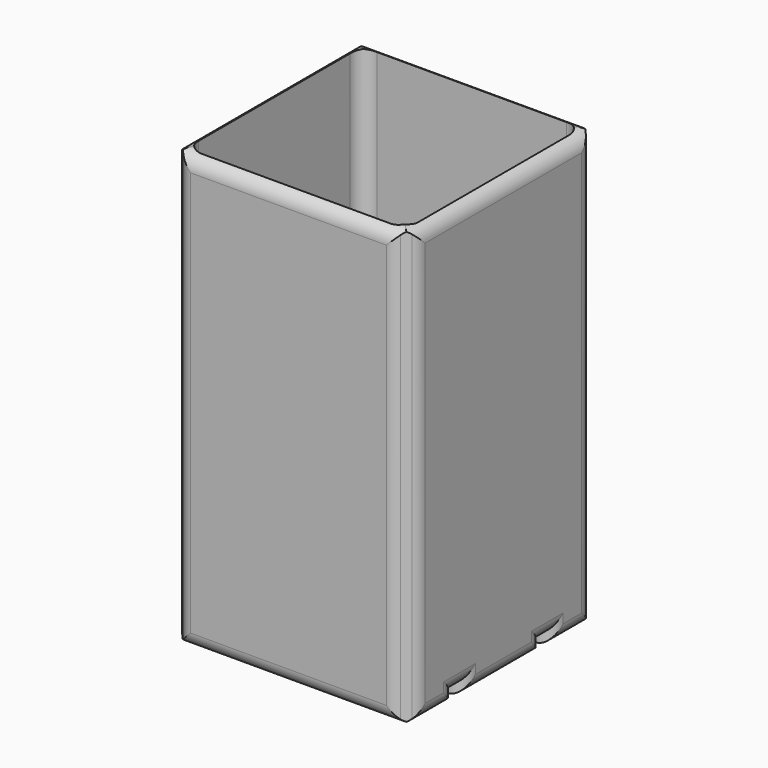
from build123d import *

# Parameters (mm, degrees)
F0_W         = 80.0557104707
F0_H         = 80.0557104707
F0_W_2       = 73.7057104707
F0_H_2       = 73.7057104707
F0_W_3       = 39.99992
F0_H_3       = 39.99992
F1_DEPTH     = 6.35
F2_DEPTH     = 9.144
F3_DEPTH     = 139.7
F4_W         = 20.0278952353
F4_H         = 3.175
F5_DEPTH     = 3.175
F6_SIZE      = 5.08
F7_T1_DEPTH  = 95.2957104707
F7_T3_DEPTH  = 156.5710244843
F7_T5_DEPTH  = 95.2957104707
F7_T7_DEPTH  = 40.3478952353
F7_T9_DEPTH  = 40.3478952353
F7_T11_DEPTH = 15.875
F7_T13_DEPTH = 3.175
F7_T15_DEPTH = 3.175
F7_T17_DEPTH = 59.04992
F7_T23_DEPTH = 28.575
F7_T27_DEPTH = 15.875
F7_T34_DEPTH = 28.575
F7_T38_DEPTH = 15.875
F7_T45_DEPTH = 15.875
F7_T49_DEPTH = 28.575
F7_T56_DEPTH = 15.875
F7_T60_DEPTH = 28.575
F8_R         = 5.08


# Not quite as in the source:
# - a fillet or chamfer that OpenCascade refuses, or shapes differently, is made with other operations: its cross-section is extruded or revolved along the edge and cut away or added


with BuildPart() as f1:
    # F0 (on Top) → F1 (new body)
    with BuildSketch(Plane.XY):
        Rectangle(F0_W, F0_H)
        Rectangle(F0_W_2, F0_H_2, mode=Mode.SUBTRACT)
        Rectangle(F0_W_2, F0_H_2)
        Rectangle(F0_W_3, F0_H_3, mode=Mode.SUBTRACT)
        Rectangle(F0_W_3, F0_H_3)
    extrude(amount=-F1_DEPTH)

    # F0 (on Top) → F2 (cut)
    with BuildSketch(Plane.XY):
        Rectangle(F0_W_3, F0_H_3)
    extrude(amount=-F2_DEPTH, mode=Mode.SUBTRACT)

    # F0 (on Top) → F3 (join)
    with BuildSketch(Plane.XY):
        Rectangle(F0_W, F0_H)
        Rectangle(F0_W_2, F0_H_2, mode=Mode.SUBTRACT)
    extrude(amount=F3_DEPTH)

    # F4 (on face) → F5 (cut)
    with BuildSketch(Plane(origin=(0, 0, -6.35), x_dir=(1, 0, 0), z_dir=(0, 0, -1))):
        with Locations((30.0139076177, 18.41246)):
            Rectangle(F4_W, F4_H)
        with Locations((30.0139076177, -18.41246)):
            Rectangle(F4_W, F4_H)
    extrude(amount=-F5_DEPTH, mode=Mode.SUBTRACT)

    # F6
    f6_edges = [f1.edges().sort_by_distance(p)[0] for p in [
        (40.027855, -40.027855, 66.675),
        (-40.027855, -40.027855, 66.675),
        (-40.027855, 40.027855, 66.675),
        (40.027855, 40.027855, 66.675),
    ]]
    chamfer(f6_edges, length=F6_SIZE)

    # F7: fillet of radius 5.08 on 24 edges, made by hand

    # F7_s2 → F7_t1 (cut)
    with BuildSketch(Plane.XZ.offset(-47.6478552353)):
        with BuildLine():
            ThreePointArc((-34.9478552353, -6.35), (-38.5399576838, -4.8621024484), (-40.0278552353, -1.27))
            Line((-40.0278552353, -1.27), (-40.0278552353, -6.35))
            Line((-40.0278552353, -6.35), (-34.9478552353, -6.35))
        make_face()
        with BuildLine():
            ThreePointArc((-34.9478552353, 139.7), (-38.5399576838, 138.2121024484), (-40.0278552353, 134.62))
            Line((-40.0278552353, 134.62), (-40.0278552353, 139.7))
            Line((-40.0278552353, 139.7), (-34.9478552353, 139.7))
        make_face()
        with BuildLine():
            ThreePointArc((40.0278552353, 134.62), (38.5399576838, 138.2121024484), (34.9478552353, 139.7))
            Line((34.9478552353, 139.7), (40.0278552353, 139.7))
            Line((40.0278552353, 139.7), (40.0278552353, 134.62))
        make_face()
    extrude(amount=F7_T1_DEPTH, mode=Mode.SUBTRACT)

    # F7_s4 → F7_t3 (cut)
    with BuildSketch(Plane.XY.offset(-11.6105122421)):
        with BuildLine():
            ThreePointArc((-38.5399576838, 36.4357527869), (-39.6411632605, 34.7876821749), (-40.0278552353, 32.8436503385))
            Line((-40.0278552353, 32.8436503385), (-40.0278552353, 34.9478552353))
            Line((-40.0278552353, 34.9478552353), (-38.5399576838, 36.4357527869))
        make_face()
        with BuildLine():
            ThreePointArc((-38.5399576838, -36.4357527869), (-39.6411632605, -34.7876821749), (-40.0278552353, -32.8436503385))
            Line((-40.0278552353, -32.8436503385), (-40.0278552353, -34.9478552353))
            Line((-40.0278552353, -34.9478552353), (-38.5399576838, -36.4357527869))
        make_face()
        with BuildLine():
            ThreePointArc((36.4357527869, 38.5399576838), (34.7876821749, 39.6411632605), (32.8436503385, 40.0278552353))
            Line((32.8436503385, 40.0278552353), (34.9478552353, 40.0278552353))
            Line((34.9478552353, 40.0278552353), (36.4357527869, 38.5399576838))
        make_face()
        with BuildLine():
            ThreePointArc((-32.8436503385, 40.0278552353), (-34.7876821749, 39.6411632605), (-36.4357527869, 38.5399576838))
            Line((-36.4357527869, 38.5399576838), (-34.9478552353, 40.0278552353))
            Line((-34.9478552353, 40.0278552353), (-32.8436503385, 40.0278552353))
        make_face()
        with BuildLine():
            ThreePointArc((40.0278552353, -32.8436503385), (39.6411632605, -34.7876821749), (38.5399576838, -36.4357527869))
            Line((38.5399576838, -36.4357527869), (40.0278552353, -34.9478552353))
            Line((40.0278552353, -34.9478552353), (40.0278552353, -32.8436503385))
        make_face()
        with BuildLine():
            ThreePointArc((40.0278552353, 32.8436503385), (39.6411632605, 34.7876821749), (38.5399576838, 36.4357527869))
            Line((38.5399576838, 36.4357527869), (40.0278552353, 34.9478552353))
            Line((40.0278552353, 34.9478552353), (40.0278552353, 32.8436503385))
        make_face()
        with BuildLine():
            ThreePointArc((-32.8436503385, -40.0278552353), (-34.7876821749, -39.6411632605), (-36.4357527869, -38.5399576838))
            Line((-36.4357527869, -38.5399576838), (-34.9478552353, -40.0278552353))
            Line((-34.9478552353, -40.0278552353), (-32.8436503385, -40.0278552353))
        make_face()
        with BuildLine():
            ThreePointArc((36.4357527869, -38.5399576838), (34.7876821749, -39.6411632605), (32.8436503385, -40.0278552353))
            Line((32.8436503385, -40.0278552353), (34.9478552353, -40.0278552353))
            Line((34.9478552353, -40.0278552353), (36.4357527869, -38.5399576838))
        make_face()
    extrude(amount=F7_T3_DEPTH, mode=Mode.SUBTRACT)

    # F7_s6 → F7_t5 (cut)
    with BuildSketch(Plane.YZ.offset(-47.6478552353)):
        with BuildLine():
            ThreePointArc((34.9478552353, -6.35), (38.5399576838, -4.8621024484), (40.0278552353, -1.27))
            Line((40.0278552353, -1.27), (40.0278552353, -6.35))
            Line((40.0278552353, -6.35), (34.9478552353, -6.35))
        make_face()
        with BuildLine():
            ThreePointArc((34.9478552353, 139.7), (38.5399576838, 138.2121024484), (40.0278552353, 134.62))
            Line((40.0278552353, 134.62), (40.0278552353, 139.7))
            Line((40.0278552353, 139.7), (34.9478552353, 139.7))
        make_face()
        with BuildLine():
            ThreePointArc((-34.9478552353, -6.35), (-38.5399576838, -4.8621024484), (-40.0278552353, -1.27))
            Line((-40.0278552353, -1.27), (-40.0278552353, -6.35))
            Line((-40.0278552353, -6.35), (-34.9478552353, -6.35))
        make_face()
        with BuildLine():
            ThreePointArc((-34.9478552353, 139.7), (-38.5399576838, 138.2121024484), (-40.0278552353, 134.62))
            Line((-40.0278552353, 134.62), (-40.0278552353, 139.7))
            Line((-40.0278552353, 139.7), (-34.9478552353, 139.7))
        make_face()
    extrude(amount=F7_T5_DEPTH, mode=Mode.SUBTRACT)

    # F7_s8 → F7_t7 (cut)
    with BuildSketch(Plane.XZ.offset(7.29996)):
        with BuildLine():
            ThreePointArc((40.0278552353, -1.27), (38.5399576838, -4.8621024484), (34.9478552353, -6.35))
            Line((34.9478552353, -6.35), (40.0278552353, -6.35))
            Line((40.0278552353, -6.35), (40.0278552353, -1.27))
        make_face()
    extrude(amount=F7_T7_DEPTH, mode=Mode.SUBTRACT)

    # F7_s10 → F7_t9 (cut)
    with BuildSketch(Plane.XZ.offset(-47.6478552353)):
        with BuildLine():
            ThreePointArc((40.0278552353, -1.27), (38.5399576838, -4.8621024484), (34.9478552353, -6.35))
            Line((34.9478552353, -6.35), (40.0278552353, -6.35))
            Line((40.0278552353, -6.35), (40.0278552353, -1.27))
        make_face()
    extrude(amount=F7_T9_DEPTH, mode=Mode.SUBTRACT)

    # F7_s12 → F7_t11 (cut)
    with BuildSketch(Plane.XY.offset(-19.05)):
        with BuildLine():
            ThreePointArc((40.0278552353, -25.07996), (38.5399576838, -21.4878575516), (34.9478552353, -19.99996))
            Line((34.9478552353, -19.99996), (40.0278552353, -19.99996))
            Line((40.0278552353, -19.99996), (40.0278552353, -25.07996))
        make_face()
        with BuildLine():
            ThreePointArc((40.0278552353, 25.07996), (38.5399576838, 21.4878575516), (34.9478552353, 19.99996))
            Line((34.9478552353, 19.99996), (40.0278552353, 19.99996))
            Line((40.0278552353, 19.99996), (40.0278552353, 25.07996))
        make_face()
        with BuildLine():
            ThreePointArc((40.0278552353, -11.74496), (38.5399576838, -15.3370624484), (34.9478552353, -16.82496))
            Line((34.9478552353, -16.82496), (40.0278552353, -16.82496))
            Line((40.0278552353, -16.82496), (40.0278552353, -11.74496))
        make_face()
        with BuildLine():
            ThreePointArc((40.0278552353, 11.74496), (38.5399576838, 15.3370624484), (34.9478552353, 16.82496))
            Line((34.9478552353, 16.82496), (40.0278552353, 16.82496))
            Line((40.0278552353, 16.82496), (40.0278552353, 11.74496))
        make_face()
    extrude(amount=F7_T11_DEPTH, mode=Mode.SUBTRACT)

    # F7_s14 → F7_t13 (cut)
    with BuildSketch(Plane.XZ.offset(16.82496)):
        with BuildLine():
            ThreePointArc((40.0278552353, 1.905), (38.5399576838, -1.6871024484), (34.9478552353, -3.175))
            Line((34.9478552353, -3.175), (40.0278552353, -3.175))
            Line((40.0278552353, -3.175), (40.0278552353, 1.905))
        make_face()
    extrude(amount=F7_T13_DEPTH, mode=Mode.SUBTRACT)

    # F7_s16 → F7_t15 (cut)
    with BuildSketch(Plane.XZ.offset(-19.99996)):
        with BuildLine():
            ThreePointArc((40.0278552353, 1.905), (38.5399576838, -1.6871024484), (34.9478552353, -3.175))
            Line((34.9478552353, -3.175), (40.0278552353, -3.175))
            Line((40.0278552353, -3.175), (40.0278552353, 1.905))
        make_face()
    extrude(amount=F7_T15_DEPTH, mode=Mode.SUBTRACT)

    # F7_s18 → F7_t17 (cut)
    with BuildSketch(Plane.XZ.offset(-29.52496)):
        with BuildLine():
            ThreePointArc((40.0278552353, -1.27), (38.5399576838, -4.8621024484), (34.9478552353, -6.35))
            Line((34.9478552353, -6.35), (40.0278552353, -6.35))
            Line((40.0278552353, -6.35), (40.0278552353, -1.27))
        make_face()
    extrude(amount=F7_T17_DEPTH, mode=Mode.SUBTRACT)


with BuildPart() as f7_tool21:
    # F7_s22 → F7_t23 (new body)
    with BuildSketch(Plane.XY.offset(-19.05)):
        with BuildLine():
            ThreePointArc((40.0278552353, -25.07996), (38.5399576838, -21.4878575516), (34.9478552353, -19.99996))
            Line((34.9478552353, -19.99996), (40.0278552353, -19.99996))
            Line((40.0278552353, -19.99996), (40.0278552353, -25.07996))
        make_face()
    extrude(amount=F7_T23_DEPTH)

    split(bisect_by=Plane.XY.offset(-3.175), keep=Keep.TOP)


with BuildPart() as f7_tool25:
    # F7_s26 → F7_t27 (new body)
    with BuildSketch(Plane.XZ.offset(16.82496)):
        with BuildLine():
            ThreePointArc((40.0278552353, 1.905), (38.5399576838, -1.6871024484), (34.9478552353, -3.175))
            Line((34.9478552353, -3.175), (40.0278552353, -3.175))
            Line((40.0278552353, -3.175), (40.0278552353, 1.905))
        make_face()
    extrude(amount=F7_T27_DEPTH)

    split(bisect_by=Plane.XZ.offset(19.99996), keep=Keep.TOP)


with BuildPart() as f7_tool21_1:
    add(f7_tool21.part)

    # F7_t29: intersect F7_tool25
    add(f7_tool25.part, mode=Mode.INTERSECT)


with BuildPart() as f1_1:
    add(f1.part)

    # F7_t19: cut F7_tool21
    add(f7_tool21_1.part, mode=Mode.SUBTRACT)


with BuildPart() as f7_tool32:
    # F7_s33 → F7_t34 (new body)
    with BuildSketch(Plane.XY.offset(-19.05)):
        with BuildLine():
            ThreePointArc((40.0278552353, 25.07996), (38.5399576838, 21.4878575516), (34.9478552353, 19.99996))
            Line((34.9478552353, 19.99996), (40.0278552353, 19.99996))
            Line((40.0278552353, 19.99996), (40.0278552353, 25.07996))
        make_face()
    extrude(amount=F7_T34_DEPTH)

    split(bisect_by=Plane.XY.offset(-3.175), keep=Keep.TOP)


with BuildPart() as f7_tool36:
    # F7_s37 → F7_t38 (new body)
    with BuildSketch(Plane.XZ.offset(-32.69996)):
        with BuildLine():
            ThreePointArc((40.0278552353, 1.905), (38.5399576838, -1.6871024484), (34.9478552353, -3.175))
            Line((34.9478552353, -3.175), (40.0278552353, -3.175))
            Line((40.0278552353, -3.175), (40.0278552353, 1.905))
        make_face()
    extrude(amount=F7_T38_DEPTH)

    split(bisect_by=Plane.XZ.offset(-19.99996), keep=Keep.BOTTOM)


with BuildPart() as f7_tool32_1:
    add(f7_tool32.part)

    # F7_t40: intersect F7_tool36
    add(f7_tool36.part, mode=Mode.INTERSECT)


with BuildPart() as f1_2:
    add(f1_1.part)

    # F7_t30: cut F7_tool32
    add(f7_tool32_1.part, mode=Mode.SUBTRACT)


with BuildPart() as f7_tool43:
    # F7_s44 → F7_t45 (new body)
    with BuildSketch(Plane.XZ.offset(4.12496)):
        with BuildLine():
            ThreePointArc((40.0278552353, 1.905), (38.5399576838, -1.6871024484), (34.9478552353, -3.175))
            Line((34.9478552353, -3.175), (40.0278552353, -3.175))
            Line((40.0278552353, -3.175), (40.0278552353, 1.905))
        make_face()
    extrude(amount=F7_T45_DEPTH)

    split(bisect_by=Plane.XZ.offset(16.82496), keep=Keep.BOTTOM)


with BuildPart() as f7_tool47:
    # F7_s48 → F7_t49 (new body)
    with BuildSketch(Plane.XY.offset(-19.05)):
        with BuildLine():
            ThreePointArc((40.0278552353, -11.74496), (38.5399576838, -15.3370624484), (34.9478552353, -16.82496))
            Line((34.9478552353, -16.82496), (40.0278552353, -16.82496))
            Line((40.0278552353, -16.82496), (40.0278552353, -11.74496))
        make_face()
    extrude(amount=F7_T49_DEPTH)

    split(bisect_by=Plane.XY.offset(-3.175), keep=Keep.TOP)


with BuildPart() as f7_tool43_1:
    add(f7_tool43.part)

    # F7_t51: intersect F7_tool47
    add(f7_tool47.part, mode=Mode.INTERSECT)


with BuildPart() as f1_3:
    add(f1_2.part)

    # F7_t41: cut F7_tool43
    add(f7_tool43_1.part, mode=Mode.SUBTRACT)


with BuildPart() as f7_tool54:
    # F7_s55 → F7_t56 (new body)
    with BuildSketch(Plane.XZ.offset(-19.99996)):
        with BuildLine():
            ThreePointArc((40.0278552353, 1.905), (38.5399576838, -1.6871024484), (34.9478552353, -3.175))
            Line((34.9478552353, -3.175), (40.0278552353, -3.175))
            Line((40.0278552353, -3.175), (40.0278552353, 1.905))
        make_face()
    extrude(amount=F7_T56_DEPTH)

    split(bisect_by=Plane.XZ.offset(-16.82496), keep=Keep.TOP)


with BuildPart() as f7_tool58:
    # F7_s59 → F7_t60 (new body)
    with BuildSketch(Plane.XY.offset(-19.05)):
        with BuildLine():
            ThreePointArc((40.0278552353, 11.74496), (38.5399576838, 15.3370624484), (34.9478552353, 16.82496))
            Line((34.9478552353, 16.82496), (40.0278552353, 16.82496))
            Line((40.0278552353, 16.82496), (40.0278552353, 11.74496))
        make_face()
    extrude(amount=F7_T60_DEPTH)

    split(bisect_by=Plane.XY.offset(-3.175), keep=Keep.TOP)


with BuildPart() as f7_tool54_1:
    add(f7_tool54.part)

    # F7_t62: intersect F7_tool58
    add(f7_tool58.part, mode=Mode.INTERSECT)


with BuildPart() as f1_4:
    add(f1_3.part)

    # F7_t52: cut F7_tool54
    add(f7_tool54_1.part, mode=Mode.SUBTRACT)

    # F8
    f8_edges = [f1_4.edges().sort_by_distance(p)[0] for p in [
        (36.852855, 36.852855, 69.664643),
        (36.852855, -36.852855, 69.664643),
        (-36.852855, -36.852855, 69.664643),
        (-36.852855, 36.852855, 69.664643),
    ]]
    fillet(f8_edges, radius=F8_R)


solid = f1_4.part
